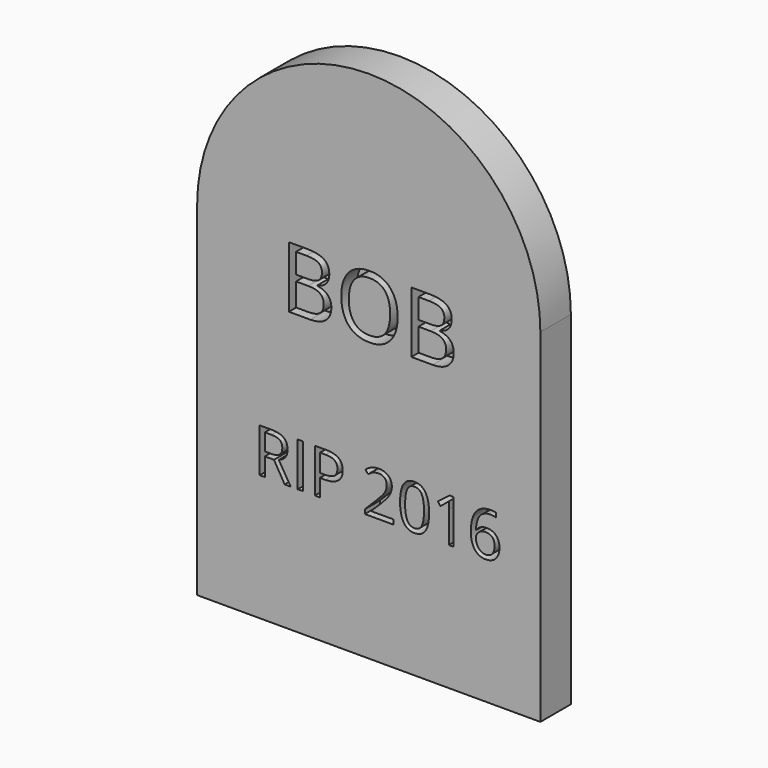
from build123d import *

# Parameters (mm, degrees)
F0_W           = 914.4
F0_H           = 914.4
F1_DEPTH       = 101.6
F2_TEXT_SIZE   = 228.5709811582
F2_TEXT_SIZE_2 = 163.8091686699
F3_DEPTH       = 50.8


# Not quite as in the source:
# - Text() gives the source's letters only with a copy of the font that has no kerning and outlines rounded to 1/6400 em; it was checked with that copy


with BuildPart() as f1:
    # F0 (on Front) → F1 (new body)
    with BuildSketch(Plane.XZ):
        with BuildLine():
            ThreePointArc((11.656133458, 919.0048923396), (-445.543866542, 1376.2048923396), (-902.743866542, 919.0048923396))
            Line((-902.743866542, 919.0048923396), (11.656133458, 919.0048923396))
        make_face()
        with Locations((-445.543866542, 461.8048923396)):
            Rectangle(F0_W, F0_H)
    extrude(amount=F1_DEPTH)

    # F2 (on face) → F3 (cut)
    with BuildSketch(Plane.XZ.offset(101.6)):
        with Locations((-680.6999146938, 748.7450242043)):
            Text('BOB', F2_TEXT_SIZE, font='Open Sans', text_align=(TextAlign.LEFT, TextAlign.BOTTOM))
        with Locations((-752.0140111446, 340.0602638721)):
            Text('RIP 2016', F2_TEXT_SIZE_2, font='Open Sans', text_align=(TextAlign.LEFT, TextAlign.BOTTOM))
    extrude(amount=-F3_DEPTH, mode=Mode.SUBTRACT)


solid = f1.part
